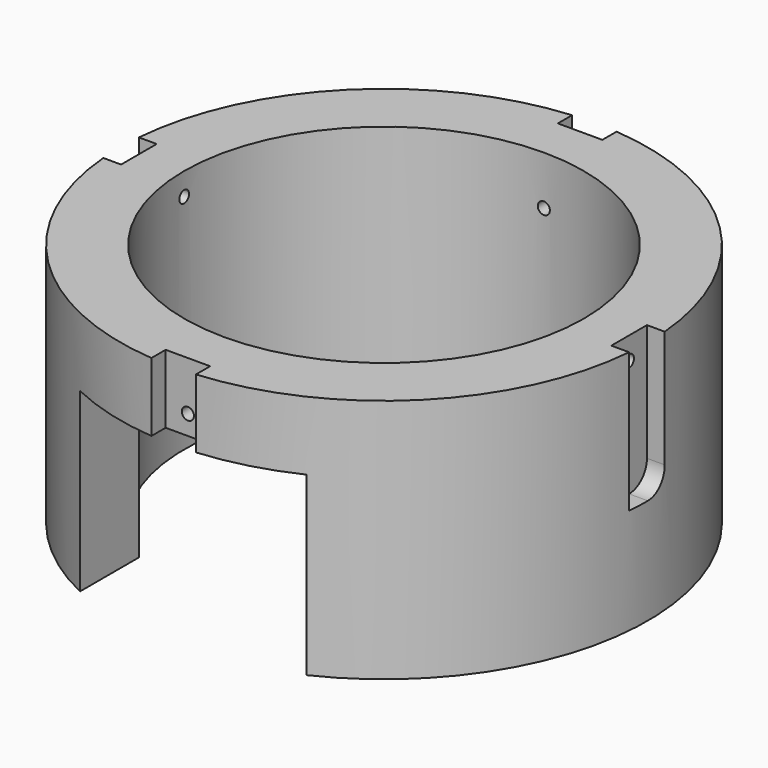
from build123d import *

# Parameters (mm, degrees)
F0_R           = 34.985
F0_R_2         = 26.5
F1_DEPTH       = 32.5
F3_DEPTH       = 23.4
F5_DEPTH       = 18.5
F6_R           = 2.95
F7_R           = 0.8
F8_DEPTH       = 34.9860001
F8_DEPTH_BACK  = 34.9860001
F10_DEPTH      = 9.4
F11_R          = 2.949
F12_R          = 0.8
F13_DEPTH      = 34.9860001
F13_DEPTH_BACK = 34.861403497


# Not quite as in the source:
# - a fillet or chamfer is up to 0.001 mm smaller than in the source, because OpenCascade refuses the exact size


with BuildPart() as f1:
    # F0 (on Top) → F1 (new body)
    with BuildSketch(Plane.XY):
        Circle(F0_R)
        Circle(F0_R_2, mode=Mode.SUBTRACT)
    extrude(amount=F1_DEPTH)

    # F2 (on face) → F3 (cut)
    with BuildSketch(Plane(origin=(0, 0, 0), x_dir=(1, 0, 0), z_dir=(0, 0, -1))):
        with BuildLine():
            ThreePointArc((15.025, 31.5942969537), (0, 34.985), (-15.025, 31.5942969537))
            Line((-15.025, 31.5942969537), (-15.025, 21.828865637))
            ThreePointArc((-15.025, 21.828865637), (0, 26.5), (15.025, 21.828865637))
            Line((15.025, 21.828865637), (15.025, 31.5942969537))
        make_face()
    extrude(amount=-F3_DEPTH, mode=Mode.SUBTRACT)

    # F4 (on face) → F5 (cut)
    with BuildSketch(Plane.XY.offset(32.5)):
        with BuildLine():
            ThreePointArc((34.985, 0), (34.9538369699, 1.4763150336), (34.860403397, 2.95))
            Line((34.860403397, 2.95), (32.5, 2.95))
            Line((32.5, 2.95), (32.5, -2.95))
            Line((32.5, -2.95), (34.860403397, -2.95))
            ThreePointArc((34.860403397, -2.95), (34.9538369699, -1.4763150336), (34.985, 0))
        make_face()
        with BuildLine():
            Line((-32.5, 2.95), (-34.860403397, 2.95))
            ThreePointArc((-34.860403397, 2.95), (-34.985, 0), (-34.860403397, -2.95))
            Line((-34.860403397, -2.95), (-32.5, -2.95))
            Line((-32.5, -2.95), (-32.5, 2.95))
        make_face()
    extrude(amount=-F5_DEPTH, mode=Mode.SUBTRACT)

    # F6
    f6_edges = [f1.edges().sort_by_distance(p)[0] for p in [
        (-33.680202, -2.95, 14),
        (33.680202, 2.95, 14),
    ]]
    fillet(f6_edges, radius=F6_R)

    # F7 (on Right) → F8 (cut, two sides)
    with BuildSketch(Plane.YZ) as f8_sk:
        with Locations((0, 29.5)):
            Circle(F7_R)
    extrude(amount=-F8_DEPTH, mode=Mode.SUBTRACT)
    extrude(f8_sk.sketch, amount=F8_DEPTH_BACK, mode=Mode.SUBTRACT)

    # F9 (on face) → F10 (cut)
    with BuildSketch(Plane.XY.offset(32.5)):
        with BuildLine():
            ThreePointArc((2.95, 34.860403397), (0, 34.985), (-2.95, 34.860403397))
            Line((-2.95, 34.860403397), (-2.95, 32.5))
            Line((-2.95, 32.5), (2.95, 32.5))
            Line((2.95, 32.5), (2.95, 34.860403397))
        make_face()
        with BuildLine():
            Line((-2.95, -32.5), (-2.95, -34.860403397))
            ThreePointArc((-2.95, -34.860403397), (0, -34.985), (2.95, -34.860403397))
            Line((2.95, -34.860403397), (2.95, -32.5))
            Line((2.95, -32.5), (-2.95, -32.5))
        make_face()
    extrude(amount=-F10_DEPTH, mode=Mode.SUBTRACT)

    # F11 (radius 2.95 in the source; OpenCascade refuses exactly that, so slightly less here)
    f11_edges = [f1.edges().sort_by_distance(p)[0] for p in [
        (-2.95, 33.680202, 23.1),
        (2.95, 33.680202, 23.1),
    ]]
    fillet(f11_edges, radius=F11_R)

    # F12 (on Front) → F13 (cut, two sides)
    with BuildSketch(Plane.XZ) as f13_sk:
        with Locations((0, 26)):
            Circle(F12_R)
    extrude(amount=-F13_DEPTH, mode=Mode.SUBTRACT)
    extrude(f13_sk.sketch, amount=F13_DEPTH_BACK, mode=Mode.SUBTRACT)


solid = f1.part
